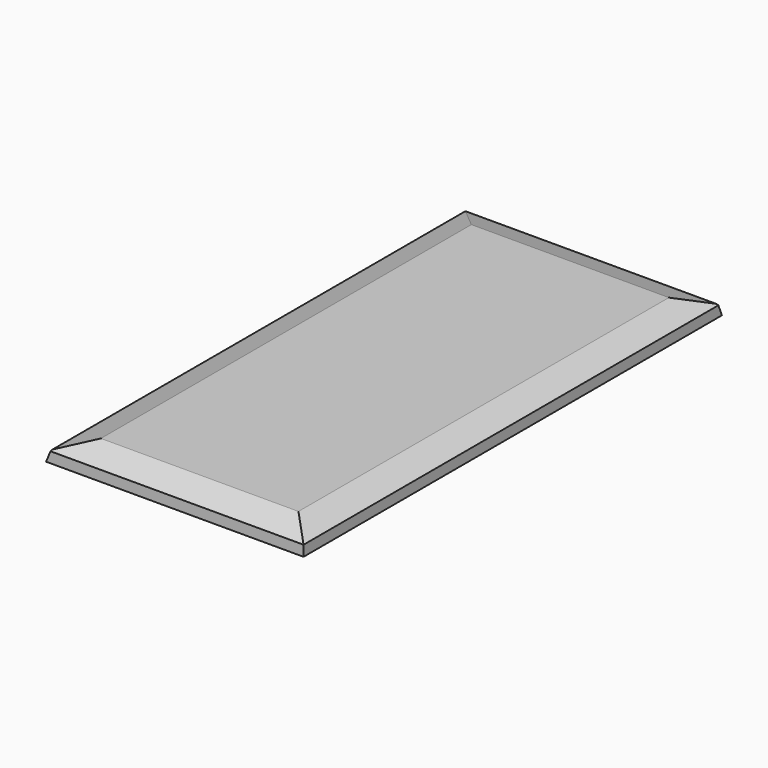
from build123d import *

# Parameters (mm, degrees)
F0_W        = 121.859960258
F0_H        = 246.6522753239
F1_DEPTH    = 10
F2_SIZE2    = 5
F2_SIZE     = 12
F3_SIZE2    = 5
F3_SIZE     = 12
F4_T1_DEPTH = 172.0821922482
F5_T1_DEPTH = 291.8745073141
F6_SIZE2    = 5
F6_SIZE     = 12
F7_SIZE2    = 5
F7_SIZE     = 12


# Not quite as in the source:
# - a fillet or chamfer that OpenCascade refuses, or shapes differently, is made with other operations: its cross-section is extruded or revolved along the edge and cut away or added


with BuildPart() as f1:
    # F0 (on Top) → F1 (new body)
    with BuildSketch(Plane.XY):
        with Locations((24.3507884443, 90.4376059771)):
            Rectangle(F0_W, F0_H)
    extrude(amount=F1_DEPTH)

    # F2
    f2_edges = [f1.edges().sort_by_distance(p)[0] for p in [
        (85.280769, 90.437606, 10),
    ]]
    f2_side = f1.faces().sort_by_distance((24.350788, 90.437606, 10))[0]
    chamfer(f2_edges, length=F2_SIZE, length2=F2_SIZE2, reference=f2_side)

    # F3
    f3_edges = [f1.edges().sort_by_distance(p)[0] for p in [
        (18.350788, -32.888532, 10),
    ]]
    f3_side = f1.faces().sort_by_distance((18.350788, 90.437606, 10))[0]
    chamfer(f3_edges, length=F3_SIZE, length2=F3_SIZE2, reference=f3_side)

    # F4: chamfer of 12 x 5 on 1 edges, made by hand

    # F4_s2 → F4_t1 (cut)
    with BuildSketch(Plane.YZ.offset(-67.6903076798)):
        Polygon((208.763743639, 10), (213.763743639, -2), (213.763743639, 10), align=None)
    extrude(amount=F4_T1_DEPTH, mode=Mode.SUBTRACT)

    # F5: chamfer of 12 x 5 on 1 edges, made by hand

    # F5_s2 → F5_t1 (cut)
    with BuildSketch(Plane.XZ.offset(-239.8748596341)):
        Polygon((-36.5791916847, -2), (-31.5791916847, 10), (-36.5791916847, 10), align=None)
    extrude(amount=F5_T1_DEPTH, mode=Mode.SUBTRACT)

    # F6
    f6_edges = [f1.edges().sort_by_distance(p)[0] for p in [
        (-31.579192, 93.937606, 10),
    ]]
    f6_side = f1.faces().sort_by_distance((20.850788, 93.937606, 10))[0]
    chamfer(f6_edges, length=F6_SIZE, length2=F6_SIZE2, reference=f6_side)

    # F7
    f7_edges = [f1.edges().sort_by_distance(p)[0] for p in [
        (26.850788, 208.763744, 10),
    ]]
    f7_side = f1.faces().sort_by_distance((26.850788, 93.937606, 10))[0]
    chamfer(f7_edges, length=F7_SIZE, length2=F7_SIZE2, reference=f7_side)


solid = f1.part
